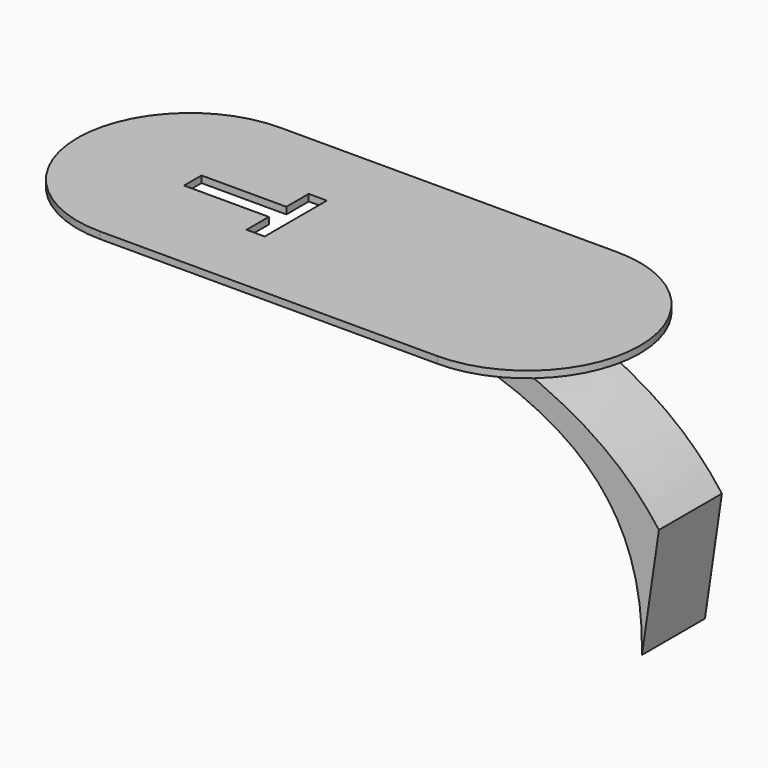
from build123d import *

# Parameters (mm, degrees)
F0_W         = 150
F0_H         = 100
F1_DEPTH     = 3
F2_W         = 82
F2_H         = 44
F2_W_2       = 74
F2_H_2       = 36
F3_DEPTH     = 4
F4_W         = 73
F4_H         = 35
F5_DEPTH     = 4
F7_DEPTH     = 35
F8_TEXT_SIZE = 64.1121963436
F9_DEPTH     = 3


# Not quite as in the source:
# - Text() gives the source's letters only with a copy of the font that has no kerning and outlines rounded to 1/6400 em; it was checked with that copy


with BuildPart() as f1:
    # F0 (on Top) → F1 (new body)
    with BuildSketch(Plane.XY):
        Rectangle(F0_W, F0_H)
        with BuildLine():
            Line((75, 50), (75, -50))
            ThreePointArc((75, -50), (125, 0), (75, 50))
        make_face()
        with BuildLine():
            ThreePointArc((-75, 50), (-125, 0), (-75, -50))
            Line((-75, -50), (-75, 50))
        make_face()
    extrude(amount=F1_DEPTH)

    # F2 (on face) → F3 (join)
    with BuildSketch(Plane(origin=(0, 0, 0), x_dir=(1, 0, 0), z_dir=(0, 0, -1))):
        with Locations((41, 0)):
            Rectangle(F2_W, F2_H)
        with Locations((41, 0)):
            Rectangle(F2_W_2, F2_H_2, mode=Mode.SUBTRACT)
    extrude(amount=F3_DEPTH)

    # F8 (on face) → F9 (cut, through all)
    with BuildSketch(Plane.XY.offset(3)):
        with Locations(Location((-73.7582332425, 18.5839472312), (0, 0, -90))):
            Text('T', F8_TEXT_SIZE, font='Open Sans', font_style=FontStyle.BOLD, text_align=(TextAlign.LEFT, TextAlign.BOTTOM))
    extrude(amount=-F9_DEPTH, mode=Mode.SUBTRACT)


with BuildPart() as f5:
    # F4 (on face) → F5 (new body)
    with BuildSketch(Plane(origin=(0, 0, 0), x_dir=(1, 0, 0), z_dir=(0, 0, -1))):
        with Locations((41, 0)):
            Rectangle(F4_W, F4_H)
    extrude(amount=F5_DEPTH)

    # F6 (on face) → F7 (join, through all)
    with BuildSketch(Plane.XZ.offset(17.5)):
        with BuildLine():
            Line((66.21055305, -4), (19.5061601698, -4))
            add(Edge.make_bspline(
                [(19.5061601698, -4), (82.3952555656, -16.8449934572), (141.4747238159, -29.3859243393), (139.8598104715, -106.0523241758)],
                knots=[0, 0, 0, 0, 157.7963181149, 157.7963181149, 157.7963181149, 157.7963181149], degree=3))
            Line((139.8598104715, -106.0523241758), (147.4043577909, -54.6774864197))
            add(Edge.make_bspline(
                [(66.21055305, -4), (100.6999611855, -15.1583747938), (127.6448071003, -28.0919019133), (147.4043577909, -54.6774864197)],
                knots=[0, 0, 0, 0, 95.7112405004, 95.7112405004, 95.7112405004, 95.7112405004], degree=3))
        make_face()
    extrude(amount=-F7_DEPTH)


solid = Compound([f1.part, f5.part])
